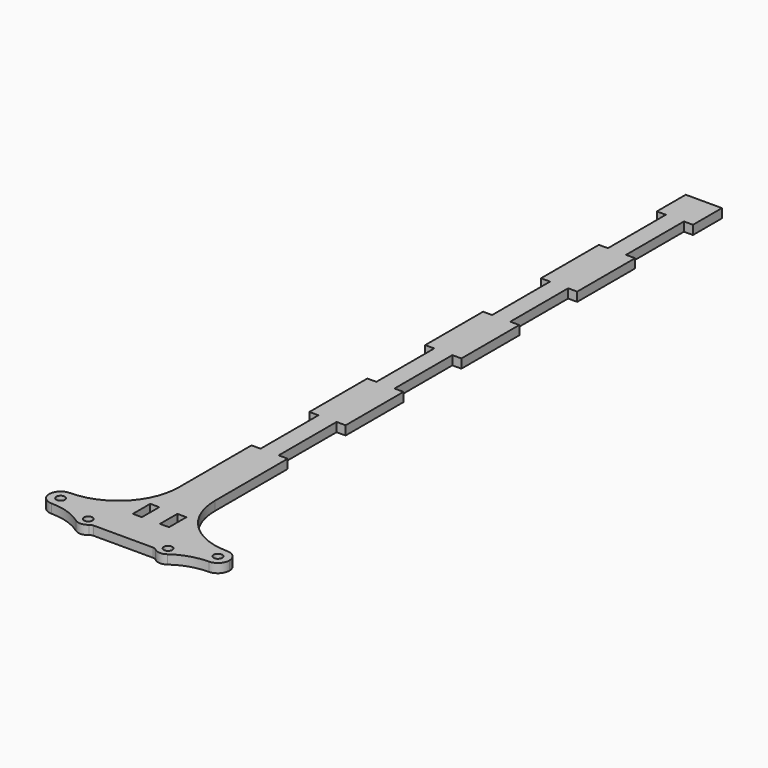
from build123d import *

# Parameters (mm, degrees)
F0_R     = 1.5
F1_DEPTH = 3.175


# Not quite as in the source:
# - a length typed as a fraction of an inch, garbled in the dataset ("3 / 203.2 mm" for 3/8 in), is restored
# - a feature names something its author has since deleted; it is built from what else it names


with BuildPart() as f1:
    # F0 (on Top) → F1 (new body)
    with BuildSketch(Plane.XY):
        with BuildLine():
            ThreePointArc((-33.3848889083, 26.7107070004), (-34.5564617835, 29.5391341252), (-37.3848889083, 30.7107070004))
            ThreePointArc((-37.3848889083, 30.7107070004), (-41.3848889083, 26.7107070004), (-37.3848889083, 22.7107070004))
            ThreePointArc((-37.3848889083, 22.7107070004), (-34.5564617835, 23.8822798757), (-33.3848889083, 26.7107070004))
        make_face()
        with Locations((-37.3848889083, 26.7107070004)):
            Circle(F0_R, mode=Mode.SUBTRACT)
        with BuildLine():
            Line((-3.4348889083, 20.3883182257), (-16.1348889083, 20.3883182257))
            Line((-16.1348889083, 20.3883182257), (-16.1348889083, 31.8183182257))
            Line((-16.1348889083, 31.8183182257), (-16.1348889083, 39.4383182257))
            Line((-16.1348889083, 39.4383182257), (-16.1348889083, 51.9607070004))
            ThreePointArc((-16.1348889083, 51.9607070004), (-22.3588698081, 36.9346879002), (-37.3848889083, 30.7107070004))
            ThreePointArc((-37.3848889083, 30.7107070004), (-34.5564617835, 29.5391341252), (-33.3848889083, 26.7107070004))
            ThreePointArc((-33.3848889083, 26.7107070004), (-34.5564617835, 23.8822798757), (-37.3848889083, 22.7107070004))
            ThreePointArc((-37.3848889083, 22.7107070004), (-31.3137586061, 21.7575229445), (-25.8268376377, 18.9896932393))
            ThreePointArc((-25.8268376377, 18.9896932393), (-25.3822585347, 24.9465327374), (-20.2848889083, 21.8323056621))
            ThreePointArc((-20.2848889083, 21.8323056621), (-20.5921773878, 20.3982229772), (-21.4600849924, 19.215955771))
            ThreePointArc((-21.4600849924, 19.215955771), (-20.8930268384, 19.5596143827), (-20.2408664312, 19.6793766243))
            Line((-20.2408664312, 19.6793766243), (0.6710886146, 19.6793766243))
            ThreePointArc((0.6710886146, 19.6793766243), (1.3232490219, 19.5596143827), (1.8903071759, 19.215955771))
            ThreePointArc((1.8903071759, 19.215955771), (2.7810284068, 25.0250171826), (7.7151110917, 21.8323056621))
            ThreePointArc((7.7151110917, 21.8323056621), (7.329338167, 20.2349360357), (6.2570598212, 18.9896932393))
            ThreePointArc((6.2570598212, 18.9896932393), (11.7439807896, 21.7575229445), (17.8151110917, 22.7107070004))
            ThreePointArc((17.8151110917, 22.7107070004), (13.8151110917, 26.7107070004), (17.8151110917, 30.7107070004))
            ThreePointArc((17.8151110917, 30.7107070004), (2.7890919915, 36.9346879002), (-3.4348889083, 51.9607070004))
            Line((-3.4348889083, 51.9607070004), (-3.4348889083, 39.4383182257))
            Line((-3.4348889083, 39.4383182257), (-3.4348889083, 31.8183182257))
            Line((-3.4348889083, 31.8183182257), (-3.4348889083, 20.3883182257))
        make_face()
        Polygon((-16.1348889083, 31.8183182257), (-16.1348889083, 20.3883182257), (-3.4348889083, 20.3883182257), (-3.4348889083, 31.8183182257), (-6.6098889083, 31.8183182257), (-6.6098889083, 39.4383182257), (-3.4348889083, 39.4383182257), (-3.4348889083, 51.9607070004), (-3.4348889083, 83.8883182257), (-6.6098889083, 83.8883182257), (-6.6098889083, 109.2883182257), (-3.4348889083, 109.2883182257), (-3.4348889083, 134.6883182257), (-6.6098889083, 134.6883182257), (-6.6098889083, 160.0883182257), (-3.4348889083, 160.0883182257), (-3.4348889083, 185.4883182257), (-6.6098889083, 185.4883182257), (-6.6098889083, 210.8883182257), (-3.4348889083, 210.8883182257), (-3.4348889083, 236.2883182257), (-6.6098889083, 236.2883182257), (-6.6098889083, 261.6883182257), (-3.4348889083, 261.6883182257), (-3.4348889083, 274.3883182257), (-16.1348889083, 274.3883182257), (-16.1348889083, 261.6883182257), (-12.9598889083, 261.6883182257), (-12.9598889083, 236.2883182257), (-16.1348889083, 236.2883182257), (-16.1348889083, 210.8883182257), (-12.9598889083, 210.8883182257), (-12.9598889083, 185.4883182257), (-16.1348889083, 185.4883182257), (-16.1348889083, 160.0883182257), (-12.9598889083, 160.0883182257), (-12.9598889083, 134.6883182257), (-16.1348889083, 134.6883182257), (-16.1348889083, 109.2883182257), (-12.9598889083, 109.2883182257), (-12.9598889083, 83.8883182257), (-16.1348889083, 83.8883182257), (-16.1348889083, 51.9607070004), (-16.1348889083, 39.4383182257), (-12.9598889083, 39.4383182257), (-12.9598889083, 31.8183182257), align=None)
        with BuildLine():
            ThreePointArc((21.8151110917, 26.7107070004), (20.6435382165, 29.5391341252), (17.8151110917, 30.7107070004))
            ThreePointArc((17.8151110917, 30.7107070004), (13.8151110917, 26.7107070004), (17.8151110917, 22.7107070004))
            ThreePointArc((17.8151110917, 22.7107070004), (20.6435382165, 23.8822798757), (21.8151110917, 26.7107070004))
        make_face()
        with Locations((17.8151110917, 26.7107070004)):
            Circle(F0_R, mode=Mode.SUBTRACT)
        with BuildLine():
            ThreePointArc((-20.2848889083, 21.8323056621), (-25.3822585347, 24.9465327374), (-25.8268376377, 18.9896932393))
            ThreePointArc((-25.8268376377, 18.9896932393), (-23.6037799702, 18.3369945812), (-21.4600849924, 19.215955771))
            ThreePointArc((-21.4600849924, 19.215955771), (-20.5921773878, 20.3982229772), (-20.2848889083, 21.8323056621))
        make_face()
        with Locations((-23.7848889083, 21.8323056621)):
            Circle(F0_R, mode=Mode.SUBTRACT)
        with BuildLine():
            ThreePointArc((1.8903071759, 19.215955771), (4.0340021537, 18.3369945812), (6.2570598212, 18.9896932393))
            ThreePointArc((6.2570598212, 18.9896932393), (7.329338167, 20.2349360357), (7.7151110917, 21.8323056621))
            ThreePointArc((7.7151110917, 21.8323056621), (2.7810284068, 25.0250171826), (1.8903071759, 19.215955771))
        make_face()
        with Locations((4.2151110917, 21.8323056621)):
            Circle(F0_R, mode=Mode.SUBTRACT)
    extrude(amount=F1_DEPTH)


solid = f1.part
